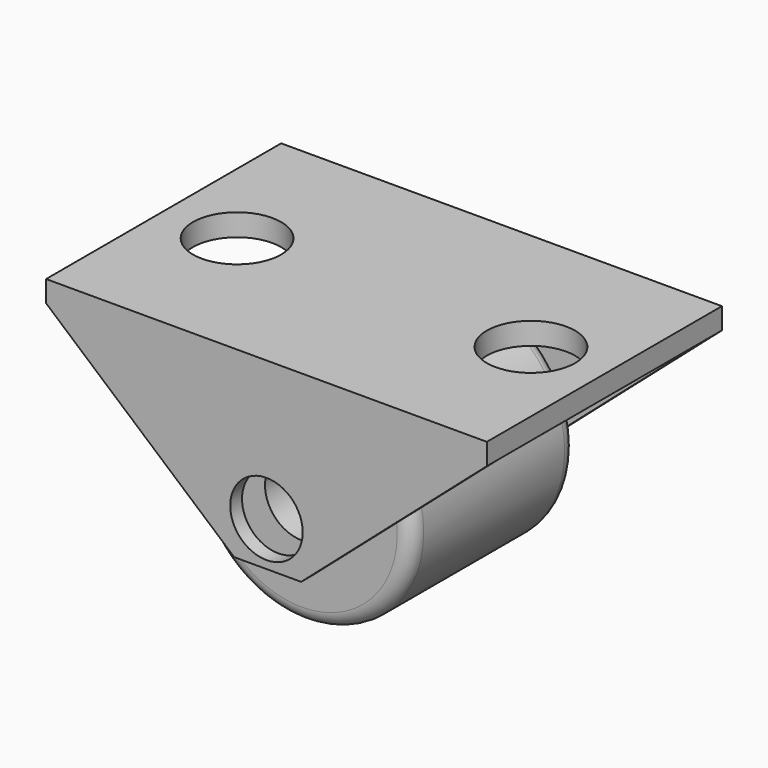
from build123d import *

# Parameters (mm, degrees)
F0_R     = 7.5
F0_R_2   = 2.5
F1_DEPTH = 7
F2_R     = 1
F3_R     = 2.4659641978
F4_DEPTH = 10
F5_W     = 32.3933225603
F5_H     = 18
F6_DEPTH = 11
F7_R     = 3
F8_DEPTH = 2


with BuildPart() as f1:
    # F0 (on Front) → F1 (new body, symmetric)
    with BuildSketch(Plane.XZ):
        Circle(F0_R)
        Circle(F0_R_2, mode=Mode.SUBTRACT)
    extrude(amount=F1_DEPTH, both=True)

    # F2
    f2_edges = [f1.edges().sort_by_distance(p)[0] for p in [
        (-7.5, -7, 0),
        (-7.5, 7, 0),
    ]]
    fillet(f2_edges, radius=F2_R)


with BuildPart() as f4:
    # F3 (on Front) → F4 (new body, symmetric)
    with BuildSketch(Plane.XZ):
        Polygon((-2.2, -3), (2.3600001695, -3), (15, 8.0461148574), (15, 9.5), (-15, 9.5), (-15, 8.0461148574), align=None)
        Circle(F3_R, mode=Mode.SUBTRACT)
    extrude(amount=F4_DEPTH, both=True)

    # F5 (on face) → F6 (cut)
    with BuildSketch(Plane(origin=(0, 0, -3), x_dir=(1, 0, 0), z_dir=(0, 0, -1))):
        Rectangle(F5_W, F5_H)
    extrude(amount=-F6_DEPTH, mode=Mode.SUBTRACT)

    # F7 (on face) → F8 (cut)
    with BuildSketch(Plane.XY.offset(9.5)):
        with Locations((-10, 0)):
            Circle(F7_R)
        with Locations((10, 0)):
            Circle(F7_R)
    extrude(amount=-F8_DEPTH, mode=Mode.SUBTRACT)


solid = Compound([f1.part, f4.part])
